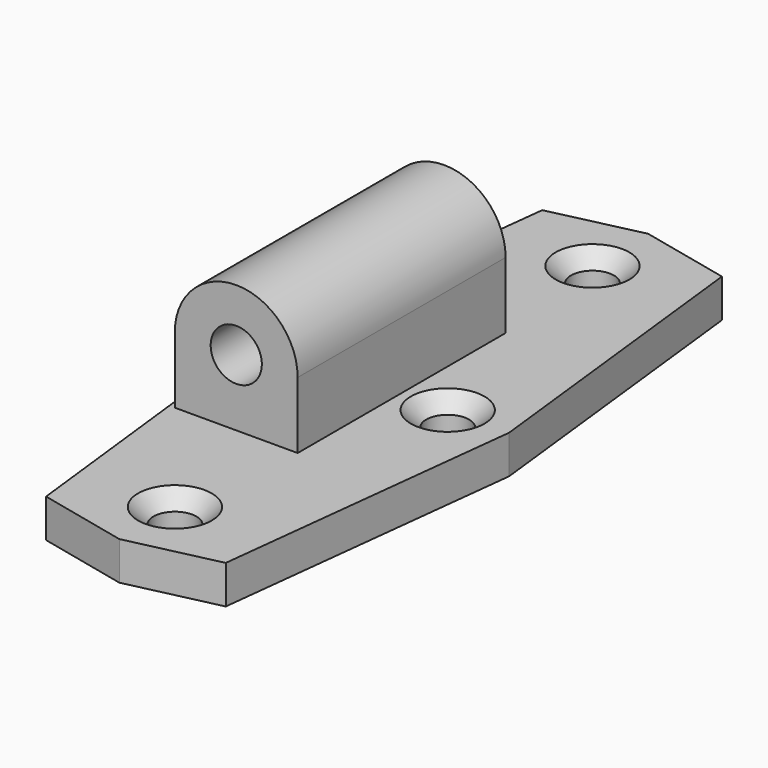
from build123d import *

# Parameters (mm, degrees)
F0_R     = 2.667
F0_W     = 15.24
F0_H     = 32.258
F1_DEPTH = 4.7625
F2_DEPTH = 13.0175
F3_W     = 7.62
F3_H     = 32.258
F6_DEPTH = 32.258
F7_SIZE  = 1.905


with BuildPart() as f1:
    # F0 (on Top) → F1 (new body)
    with BuildSketch(Plane.XY):
        Polygon((-11.1125, -38.481), (0, -41.021), (11.1834268409, -38.481), (15.5575, 0), (11.1834268409, 38.481), (0, 41.021), (-11.1125, 38.481), (-15.5575, 0), align=None)
        with Locations((0, -32.385)):
            Circle(F0_R, mode=Mode.SUBTRACT)
        with Locations((-5.3975, 0)):
            Rectangle(F0_W, F0_H, mode=Mode.SUBTRACT)
        with Locations((0, 32.385)):
            Circle(F0_R, mode=Mode.SUBTRACT)
        with Locations((7.9375, 0)):
            Circle(F0_R, mode=Mode.SUBTRACT)
    extrude(amount=F1_DEPTH)

    # F0 (on Top) → F2 (join)
    with BuildSketch(Plane.XY):
        with Locations((-5.3975, 0)):
            Rectangle(F0_W, F0_H)
    extrude(amount=F2_DEPTH)

    # F3 (on face) → F4 (revolve)
    with BuildSketch(Plane.XY.offset(13.0175)):
        with Locations((-9.2075, 0)):
            Rectangle(F3_W, F3_H)
    revolve(axis=Axis((-5.3975, 0, 13.0175), (0, -1, 0)))

    # F5 (on face) → F6 (cut)
    with BuildSketch(Plane.XZ.offset(16.129)):
        with BuildLine():
            ThreePointArc((-2.2225, 13.0175), (-5.3975, 16.1925), (-8.5725, 13.0175))
            ThreePointArc((-8.5725, 13.0175), (-5.3975, 9.8425), (-2.2225, 13.0175))
        make_face()
    extrude(amount=-F6_DEPTH, mode=Mode.SUBTRACT)

    # F7
    f7_edges = [f1.edges().sort_by_distance(p)[0] for p in [
        (-2.667, -32.385, 4.7625),
        (5.2705, 0, 4.7625),
        (-2.667, 32.385, 4.7625),
    ]]
    chamfer(f7_edges, length=F7_SIZE)


solid = f1.part
